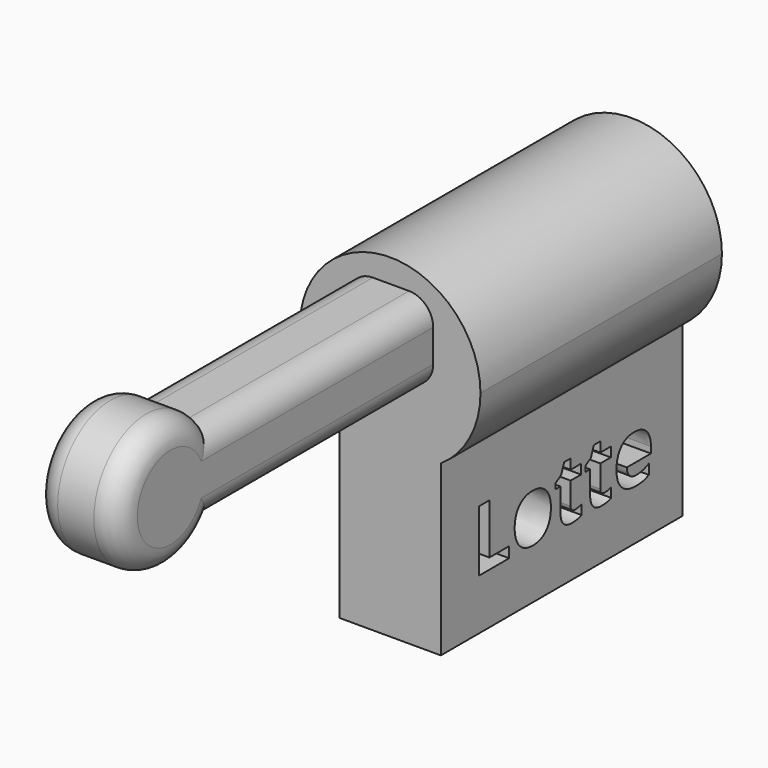
from build123d import *

# Parameters (mm, degrees)
F1_DEPTH     = 25
F2_TEXT_SIZE = 7.0890062489
F3_DEPTH     = 10
F5_DEPTH     = 3.5
F6_R         = 2


# Not quite as in the source:
# - ends of sketch curves that miss each other by under 0.0002 mm in the source are joined
# - Text() gives the source's letters only with a copy of the font that has no kerning and outlines rounded to 1/6400 em; it was checked with that copy


with BuildPart() as f1:
    # F0 (on Front) → F1 (new body)
    with BuildSketch(Plane.XZ):
        with BuildLine():
            ThreePointArc((4.1356796063, 4.6860890092), (6.5459023399, 7.3737167179), (7.4169159164, 10.8771224432))
            ThreePointArc((7.4169159164, 10.8771224432), (-3.5677259051, 17.4873448828), (-4.2643197629, 4.6860889426))
            Line((-4.2643197629, 4.6860889426), (4.1356796063, 4.6860890092))
        make_face()
        with BuildLine():
            Line((4.1356798828, 4.6860889302), (-4.2643197446, 4.6860889302))
            ThreePointArc((-4.2643197446, 4.6860889302), (-0.0643200681, 3.3958863994), (4.1356798828, 4.6860889302))
        make_face()
        with BuildLine():
            ThreePointArc((4.1356796063, 4.6860890092), (-0.0643200681, 3.3958863994), (-4.2643197629, 4.6860889426))
            Line((-4.2643197629, 4.6860889426), (-4.2643197812, -9.313911045))
            Line((-4.2643197812, -9.313911045), (4.1356798461, -9.3139110943))
            Line((4.1356798461, -9.3139110943), (4.1356796063, 4.6860890092))
        make_face()
    extrude(amount=F1_DEPTH)

    # F2 (on Right) → F3 (cut)
    with BuildSketch(Plane.YZ):
        with Locations((-21.6827467084, -5.1040844992)):
            Text('Lotte', F2_TEXT_SIZE, font='Open Sans', font_style=FontStyle.BOLD, text_align=(TextAlign.LEFT, TextAlign.BOTTOM))
        with BuildLine():
            add(Edge.make_bspline(
                [(-16.0957236585, -2.2983887447), (-16.2829177298, -2.5841643092), (-16.2829177298, -3.1623613813)],
                knots=[0, 0, 0, 1, 1, 1], degree=2))
            add(Edge.make_bspline(
                [(-16.2829177298, -3.1623613813), (-16.2829177298, -3.7372354818), (-16.0940621727, -4.0313184754)],
                knots=[0, 0, 0, 1, 1, 1], degree=2))
            add(Edge.make_bspline(
                [(-16.0940621727, -4.0313184754), (-15.9052066156, -4.325401469), (-15.4798662406, -4.325401469)],
                knots=[0, 0, 0, 1, 1, 1], degree=2))
            add(Edge.make_bspline(
                [(-15.4798662406, -4.325401469), (-15.0567411802, -4.325401469), (-14.8717624234, -4.0329799613)],
                knots=[0, 0, 0, 1, 1, 1], degree=2))
            add(Edge.make_bspline(
                [(-14.8717624234, -4.0329799613), (-14.6867836665, -3.7405584535), (-14.6867836665, -3.1623613813)],
                knots=[0, 0, 0, 1, 1, 1], degree=2))
            add(Edge.make_bspline(
                [(-14.6867836665, -3.1623613813), (-14.6867836665, -2.5874872808), (-14.8734239092, -2.3000502306)],
                knots=[0, 0, 0, 1, 1, 1], degree=2))
            add(Edge.make_bspline(
                [(-14.8734239092, -2.3000502306), (-15.0600641518, -2.0126131803), (-15.486512184, -2.0126131803)],
                knots=[0, 0, 0, 1, 1, 1], degree=2))
            add(Edge.make_bspline(
                [(-15.486512184, -2.0126131803), (-15.9085295873, -2.0126131803), (-16.0957236585, -2.2983887447)],
                knots=[0, 0, 0, 1, 1, 1], degree=2))
        make_face()
        with BuildLine():
            add(Edge.make_bspline(
                [(-4.4442772942, -2.1255942174), (-4.6414402805, -1.91292403), (-4.9770604201, -1.91292403)],
                knots=[0, 0, 0, 1, 1, 1], degree=2))
            add(Edge.make_bspline(
                [(-4.9770604201, -1.91292403), (-5.3126805597, -1.91292403), (-5.5031976026, -2.1255942174)],
                knots=[0, 0, 0, 1, 1, 1], degree=2))
            add(Edge.make_bspline(
                [(-5.5031976026, -2.1255942174), (-5.6937146455, -2.3382644049), (-5.7214060762, -2.7292674058)],
                knots=[0, 0, 0, 1, 1, 1], degree=2))
            Line((-5.7214060762, -2.7292674058), (-4.2393607073, -2.7292674058))
            add(Edge.make_bspline(
                [(-4.2393607073, -2.7292674058), (-4.2471143079, -2.3382644049), (-4.4442772942, -2.1255942174)],
                knots=[0, 0, 0, 1, 1, 1], degree=2))
        make_face()
    extrude(amount=F3_DEPTH, mode=Mode.SUBTRACT)

    # F4 (on Right) → F5 (join, symmetric)
    with BuildSketch(Plane.YZ):
        with BuildLine():
            Line((-47.9271635413, 16.4056532085), (-47.9007986667, 16.4056532085))
            ThreePointArc((-47.9007986667, 16.4056532085), (-57.6382629713, 13.0603653379), (-47.9007986667, 9.7150774673))
            Line((-47.9007986667, 9.7150774673), (-47.9271635413, 9.7150774673))
            Line((-47.9271635413, 9.7150774673), (-47.9271635413, 16.4056532085))
        make_face()
        with BuildLine():
            Line((-23.9268597215, 9.7150774673), (-23.9268597215, 16.4056532085))
            Line((-23.9268597215, 16.4056532085), (-47.9007986667, 16.4056532085))
            ThreePointArc((-47.9007986667, 16.4056532085), (-47.0468595462, 14.8289641228), (-46.7515311996, 13.0603653379))
            ThreePointArc((-46.7515311996, 13.0603653379), (-47.0468595462, 11.2917665529), (-47.9007986667, 9.7150774673))
            Line((-47.9007986667, 9.7150774673), (-23.9268597215, 9.7150774673))
        make_face()
        with BuildLine():
            ThreePointArc((-46.7515311996, 13.0603653379), (-47.0468595462, 14.8289641228), (-47.9007986667, 16.4056532085))
            Line((-47.9007986667, 16.4056532085), (-47.9271635413, 16.4056532085))
            Line((-47.9271635413, 16.4056532085), (-47.9271635413, 9.7150774673))
            Line((-47.9271635413, 9.7150774673), (-47.9007986667, 9.7150774673))
            ThreePointArc((-47.9007986667, 9.7150774673), (-47.0468595462, 11.2917665529), (-46.7515311996, 13.0603653379))
        make_face()
    extrude(amount=F5_DEPTH, both=True)

    # F6
    f6_edges = [f1.edges().sort_by_distance(p)[0] for p in [
        (-3.5, -36.450399, 16.405653),
        (-3.5, -36.450399, 9.715077),
        (3.5, -36.450399, 16.405653),
        (3.5, -36.450399, 9.715077),
        (3.5, -57.638263, 13.060365),
        (-3.5, -57.638263, 13.060365),
    ]]
    fillet(f6_edges, radius=F6_R)


solid = f1.part
